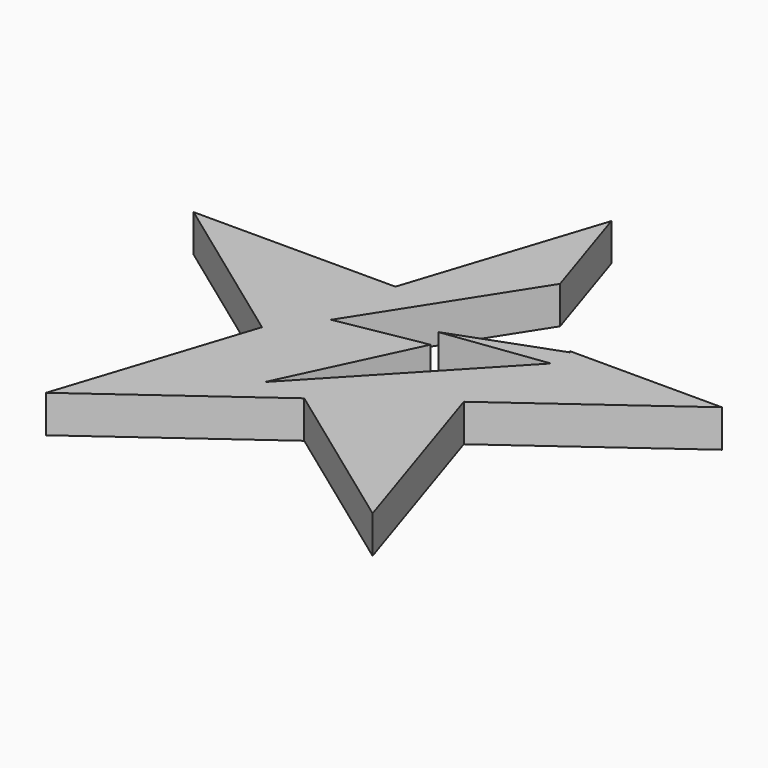
from build123d import *

# Parameters (mm, degrees)
F1_DEPTH = 7.62
F3_DEPTH = 25.4


# Not quite as in the source:
# - ends of sketch curves that miss each other by under 0.0002 mm in the source are joined


with BuildPart() as f1:
    # F0 (on Top) → F1 (new body)
    with BuildSketch(Plane.XY):
        Polygon((0, 56.5666313121), (-12.7, 17.48005039), (12.7, 17.48005039), align=None)
        Polygon((12.7, 17.48005039), (-12.7, 17.48005039), (-20.5490316571, -6.6767851239), (0, -21.6065305321), (20.5490316571, -6.6767851239), align=None)
        Polygon((-20.5490316571, -6.6767851239), (-12.7, 17.48005039), (-53.7980635454, 17.48005039), align=None)
        Polygon((53.7980636, 17.48005039), (12.7, 17.48005039), (20.5490316571, -6.6767851239), align=None)
        Polygon((0, -21.6065305321), (-20.5490316571, -6.6767851239), (-33.2490320312, -45.7633663178), align=None)
        Polygon((33.2490317454, -45.7633663178), (20.5490316571, -6.6767851239), (0, -21.6065305321), align=None)
    extrude(amount=F1_DEPTH)

    # F2 (on Top) → F3 (cut)
    with BuildSketch(Plane.XY):
        Polygon((23.131839931, 17.1561446041), (7.3025235906, 34.8562002182), (-13.5633936152, 2.1902460139), (4.1366601363, 5.3561092354), (-8.3828903735, -21.1220216006), (23.131839931, 12.2634470463), (2.4098258, 9.5292925835), align=None)
    extrude(amount=F3_DEPTH, mode=Mode.SUBTRACT)


solid = f1.part
